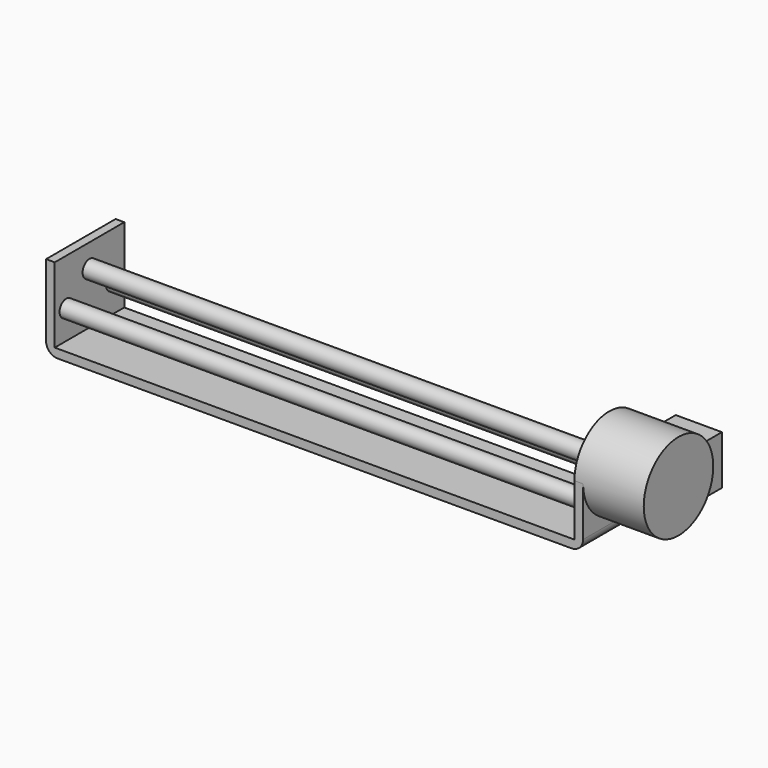
from build123d import *
from build123d import SkipClean  # not in build123d's __all__

# Parameters (mm, degrees)
F0_W           = 93
F0_H           = 15.05
F1_DEPTH       = 1.5
F2_W           = 15.05
F2_H           = 13
F3_DEPTH       = 1.5
F4_R           = 2
F6_DEPTH       = 1.5
F7_R           = 2
F9_DEPTH       = 93
F11_DEPTH      = 10.5
F13_DEPTH      = 90
F15_W          = 8
F15_H          = 8.5
F16_DEPTH      = 2.5
F16_DEPTH_BACK = 2.5


# Not quite as in the source:
# - after a boolean that leaves OpenCascade's solid faulty, fix() repairs it
# - a feature names something its author has since deleted; it is built from what else it names


with BuildPart() as f1:
    # F0 (on Top) → F1 (new body)
    with BuildSketch(Plane.XY):
        with Locations((0, -8.8193283182)):
            Rectangle(F0_W, F0_H)
    extrude(amount=F1_DEPTH)

    # F2 (on face) → F3 (join)
    with BuildSketch(Plane(origin=(-46.5, 0, 0), x_dir=(0, -1, 0), z_dir=(-1, 0, 0))):
        with Locations((8.8193283182, 8)):
            Rectangle(F2_W, F2_H)
    extrude(amount=-F3_DEPTH)

    # F4
    f4_edges = [f1.edges().sort_by_distance(p)[0] for p in [
        (-46.5, -8.819328, 0),
    ]]
    fillet(f4_edges, radius=F4_R)

    # F5 (on face) → F6 (join)
    with BuildSketch(Plane.YZ.offset(46.5)):
        with BuildLine():
            Line((-16.3443283182, 10.475), (-16.3443283182, 0))
            Line((-16.3443283182, 0), (-1.2943283182, 0))
            Line((-1.2943283182, 0), (-1.2943283182, 10.475))
            ThreePointArc((-1.2943283182, 10.475), (-8.8193283182, 2.95), (-16.3443283182, 10.475))
        make_face()
        with BuildLine():
            ThreePointArc((-1.2943283182, 10.475), (-8.8193283182, 18), (-16.3443283182, 10.475))
            Line((-16.3443283182, 10.475), (-1.2943283182, 10.475))
        make_face()
        with BuildLine():
            Line((-1.2943283182, 10.475), (-16.3443283182, 10.475))
            ThreePointArc((-16.3443283182, 10.475), (-8.8193283182, 2.95), (-1.2943283182, 10.475))
        make_face()
    extrude(amount=-F6_DEPTH)

    # F7
    f7_edges = [f1.edges().sort_by_distance(p)[0] for p in [
        (46.5, -8.819328, 0),
    ]]
    fillet(f7_edges, radius=F7_R)

    # F8 (on face) → F9 (join)
    with BuildSketch(Plane.YZ.offset(46.5)):
        with BuildLine():
            ThreePointArc((-7.3193283182, 10.475), (-8.8193283182, 11.975), (-10.3193283182, 10.475))
            Line((-10.3193283182, 10.475), (-7.3193283182, 10.475))
        make_face()
        with BuildLine():
            Line((-7.3193283182, 10.475), (-10.3193283182, 10.475))
            ThreePointArc((-10.3193283182, 10.475), (-8.8193283182, 8.975), (-7.3193283182, 10.475))
        make_face()
    extrude(amount=-F9_DEPTH)

    # F10 (on face) → F11 (join)
    with BuildSketch(Plane.YZ.offset(46.5)):
        with BuildLine():
            ThreePointArc((-1.2943283182, 10.475), (-8.8193283182, 18), (-16.3443283182, 10.475))
            Line((-16.3443283182, 10.475), (-1.2943283182, 10.475))
        make_face()
        with BuildLine():
            Line((-1.2943283182, 10.475), (-16.3443283182, 10.475))
            ThreePointArc((-16.3443283182, 10.475), (-8.8193283182, 2.95), (-1.2943283182, 10.475))
        make_face()
    with SkipClean():  # cleaning this boolean's faces spoils the solid; the shape is the same uncleaned
        extrude(amount=F11_DEPTH)

    # F12 (on face) → F13 (join, through all)
    with BuildSketch(Plane.YZ.offset(-45)):
        with BuildLine():
            ThreePointArc((-12.3893283182, 6.5), (-13.8443283182, 7.955), (-15.2993283182, 6.5))
            Line((-15.2993283182, 6.5), (-13.8443283182, 6.5))
            Line((-13.8443283182, 6.5), (-12.3893283182, 6.5))
        make_face()
        with BuildLine():
            Line((-13.8443283182, 6.5), (-15.2993283182, 6.5))
            ThreePointArc((-15.2993283182, 6.5), (-13.8443283182, 5.045), (-12.3893283182, 6.5))
            Line((-12.3893283182, 6.5), (-13.8443283182, 6.5))
        make_face()
        with BuildLine():
            ThreePointArc((-5.2493283182, 6.5), (-3.7943283182, 5.045), (-2.3393283182, 6.5))
            Line((-2.3393283182, 6.5), (-3.7943283182, 6.5))
            Line((-3.7943283182, 6.5), (-5.2493283182, 6.5))
        make_face()
        with BuildLine():
            Line((-3.7943283182, 6.5), (-2.3393283182, 6.5))
            ThreePointArc((-2.3393283182, 6.5), (-3.7943283182, 7.955), (-5.2493283182, 6.5))
            Line((-5.2493283182, 6.5), (-3.7943283182, 6.5))
        make_face()
    extrude(amount=F13_DEPTH)

    add(f1.part.fix(), mode=Mode.REPLACE)

    # F15 (on offset) → F16 (join, two sides)
    with BuildSketch(Plane(origin=(0, -1.2943283182, 0), x_dir=(-1, 0, 0), z_dir=(0, 1, 0))) as f16_sk:
        with Locations((-52.5, 10.2375)):
            Rectangle(F15_W, F15_H)
    extrude(amount=F16_DEPTH)
    extrude(f16_sk.sketch, amount=-F16_DEPTH_BACK)


solid = f1.part
